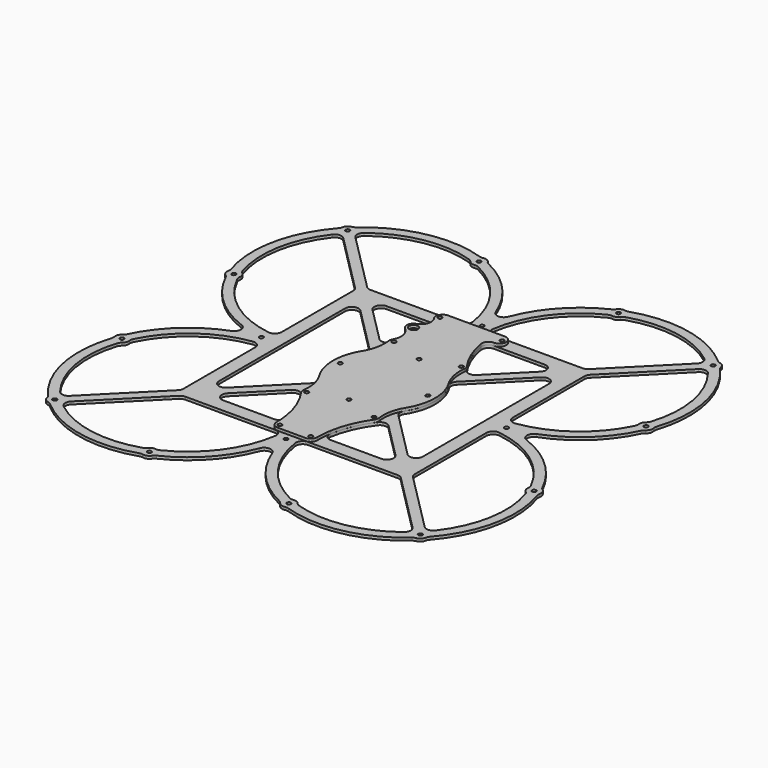
from build123d import *

# Parameters (mm, degrees)
F0_R     = 1.5
F0_W     = 52
F0_H     = 52
F1_DEPTH = 2
F2_R     = 1.5
F2_R_2   = 3.25
F3_DEPTH = 2
F4_D     = 3
F6_D     = 3


# Not quite as in the source:
# - a feature of the source that left no trace in its solid (it failed there, or was rolled back) is left out
# - a feature names something its author has since deleted; it is built from what else it names


with BuildPart() as f1:
    # F0 (on Top) → F1 (new body)
    with BuildSketch(Plane.XY):
        with BuildLine():
            ThreePointArc((-4.6783625731, -108.4060017484), (0, -105.1703496831), (4.6783625731, -108.4060017484))
            ThreePointArc((4.6783625731, -108.4060017484), (20.6623898882, -134.3994303851), (45.1726415045, -152.576202024))
            ThreePointArc((45.1726415045, -152.576202024), (46.2648777578, -153.2890175875), (47.1356036044, -154.2600595849))
            ThreePointArc((47.1356036044, -154.2600595849), (49.3956359115, -156.0747849076), (52.2827571645, -156.3307241522))
            ThreePointArc((52.2827571644, -156.3307241522), (53.5833623617, -156.2331937382), (54.8649423602, -156.4753481682))
            ThreePointArc((54.8649423602, -156.4753481682), (96.0251691017, -158.8888075411), (132.9814512389, -140.6070608479))
            ThreePointArc((132.9814512389, -140.6070608479), (134.0669737735, -139.8840623089), (135.3025491663, -139.4664027473))
            ThreePointArc((135.3025491663, -139.4664027473), (137.8609824083, -138.1042744963), (139.2338336739, -135.5515791701))
            ThreePointArc((139.2338336739, -135.5515791701), (139.656673946, -134.317767124), (140.3842208965, -133.2352877961))
            ThreePointArc((140.3842208965, -133.2352877961), (158.841500681, -96.2563147843), (156.5171132492, -54.9923735629))
            ThreePointArc((156.5171132492, -54.9923735629), (156.277094073, -53.7103919501), (156.3767909626, -52.4099510283))
            ThreePointArc((156.3767909626, -52.4099510283), (156.1256615791, -49.5224074254), (154.3147036453, -47.2593551971))
            ThreePointArc((154.3147036453, -47.2593551971), (153.3451134924, -46.38701295), (152.6341184178, -45.2935907696))
            ThreePointArc((152.6341184178, -45.2935907696), (134.44883526, -20.7077210858), (108.4060017484, -4.6783625731))
            ThreePointArc((108.4060017484, -4.6783625731), (105.1703496831, 0), (108.4060017484, 4.6783625731))
            ThreePointArc((108.4060017484, 4.6783625731), (134.44883526, 20.7077210858), (152.6341184178, 45.2935907696))
            ThreePointArc((152.6341184178, 45.2935907696), (153.3451134924, 46.38701295), (154.3147036453, 47.2593551971))
            ThreePointArc((154.3147036453, 47.2593551971), (156.1256615791, 49.5224074254), (156.3767909626, 52.4099510283))
            ThreePointArc((156.3767909626, 52.4099510283), (156.277094073, 53.7103919501), (156.5171132492, 54.9923735629))
            ThreePointArc((156.5171132492, 54.9923735629), (158.841500681, 96.2563147843), (140.3842208965, 133.2352877961))
            ThreePointArc((140.3842208965, 133.2352877961), (139.656673946, 134.317767124), (139.2338336739, 135.5515791701))
            ThreePointArc((139.2338336739, 135.5515791701), (137.8609824083, 138.1042744963), (135.3025491663, 139.4664027473))
            ThreePointArc((135.3025491663, 139.4664027473), (134.0669737735, 139.8840623089), (132.9814512389, 140.6070608479))
            ThreePointArc((132.9814512389, 140.6070608479), (96.0251691017, 158.8888075411), (54.8649423602, 156.4753481682))
            ThreePointArc((54.8649423602, 156.4753481682), (53.5833623617, 156.2331937382), (52.2827571645, 156.3307241522))
            ThreePointArc((52.2827571645, 156.3307241522), (49.3956359115, 156.0747849076), (47.1356036044, 154.2600595849))
            ThreePointArc((47.1356036044, 154.2600595849), (46.2648777578, 153.2890175875), (45.1726415045, 152.576202024))
            ThreePointArc((45.1726415045, 152.576202024), (20.6623898883, 134.3994303851), (4.6783625731, 108.4060017484))
            ThreePointArc((4.6783625731, 108.4060017484), (0, 105.1703496831), (-4.6783625731, 108.4060017484))
            ThreePointArc((-4.6783625731, 108.4060017484), (-20.6623898882, 134.3994303851), (-45.1726415045, 152.576202024))
            ThreePointArc((-45.1726415045, 152.576202024), (-46.2648777578, 153.2890175875), (-47.1356036044, 154.2600595849))
            ThreePointArc((-47.1356036044, 154.2600595849), (-49.3956359115, 156.0747849076), (-52.2827571644, 156.3307241522))
            ThreePointArc((-52.2827571644, 156.3307241522), (-53.5833623617, 156.2331937382), (-54.8649423602, 156.4753481682))
            ThreePointArc((-54.8649423602, 156.4753481682), (-96.0251691017, 158.8888075411), (-132.9814512389, 140.6070608479))
            ThreePointArc((-132.9814512389, 140.6070608479), (-134.0669737735, 139.8840623089), (-135.3025491663, 139.4664027473))
            ThreePointArc((-135.3025491663, 139.4664027473), (-137.8609824083, 138.1042744963), (-139.2338336739, 135.5515791701))
            ThreePointArc((-139.2338336739, 135.5515791701), (-139.656673946, 134.317767124), (-140.3842208964, 133.2352877961))
            ThreePointArc((-140.3842208964, 133.2352877961), (-158.841500681, 96.2563147843), (-156.5171132492, 54.9923735629))
            ThreePointArc((-156.5171132492, 54.9923735629), (-156.277094073, 53.7103919501), (-156.3767909626, 52.4099510283))
            ThreePointArc((-156.3767909626, 52.4099510283), (-156.1256615791, 49.5224074254), (-154.3147036453, 47.2593551971))
            ThreePointArc((-154.3147036453, 47.2593551971), (-153.3451134924, 46.38701295), (-152.6341184178, 45.2935907696))
            ThreePointArc((-152.6341184178, 45.2935907696), (-134.44883526, 20.7077210858), (-108.4060017484, 4.6783625731))
            ThreePointArc((-108.4060017484, 4.6783625731), (-105.1703496831, 0), (-108.4060017484, -4.6783625731))
            ThreePointArc((-108.4060017484, -4.6783625731), (-134.44883526, -20.7077210858), (-152.6341184178, -45.2935907696))
            ThreePointArc((-152.6341184178, -45.2935907696), (-153.3451134924, -46.38701295), (-154.3147036453, -47.2593551971))
            ThreePointArc((-154.3147036453, -47.2593551971), (-156.1256615791, -49.5224074254), (-156.3767909626, -52.4099510283))
            ThreePointArc((-156.3767909626, -52.4099510283), (-156.277094073, -53.7103919501), (-156.5171132492, -54.9923735629))
            ThreePointArc((-156.5171132492, -54.9923735629), (-158.841500681, -96.2563147843), (-140.3842208965, -133.2352877961))
            ThreePointArc((-140.3842208965, -133.2352877961), (-139.656673946, -134.317767124), (-139.2338336739, -135.5515791701))
            ThreePointArc((-139.2338336739, -135.5515791701), (-137.8609824083, -138.1042744963), (-135.3025491663, -139.4664027473))
            ThreePointArc((-135.3025491663, -139.4664027473), (-134.0669737735, -139.8840623089), (-132.9814512389, -140.6070608479))
            ThreePointArc((-132.9814512389, -140.6070608479), (-96.0251691017, -158.8888075411), (-54.8649423602, -156.4753481682))
            ThreePointArc((-54.8649423602, -156.4753481682), (-53.5833623617, -156.2331937382), (-52.2827571644, -156.3307241522))
            ThreePointArc((-52.2827571644, -156.3307241522), (-49.3956359115, -156.0747849076), (-47.1356036044, -154.2600595849))
            ThreePointArc((-47.1356036044, -154.2600595849), (-46.2648777578, -153.2890175875), (-45.1726415045, -152.576202024))
            ThreePointArc((-45.1726415045, -152.576202024), (-20.6623898883, -134.3994303851), (-4.6783625731, -108.4060017484))
        make_face()
        with Locations((-134.3328737249, -134.5613309295)):
            Circle(F0_R, mode=Mode.SUBTRACT)
        with Locations((-51.261755673, -151.4360785108)):
            Circle(F0_R, mode=Mode.SUBTRACT)
        with BuildLine():
            Line((-63.8445055786, -85), (-12.2338580115, -85))
            ThreePointArc((-12.2338580115, -85), (-8.449043945, -86.7327102238), (-7.2874242898, -90.7299270073))
            ThreePointArc((-7.2874242898, -90.7299270073), (-20.6592480643, -123.369634074), (-47.6974444383, -146.0211701213))
            ThreePointArc((-47.6974444383, -146.0211701213), (-49.1034491788, -146.4668977038), (-50.5783264353, -146.4830062847))
            ThreePointArc((-50.5783264353, -146.4830062847), (-53.1278754345, -146.797372114), (-55.1848415227, -148.3361757032))
            ThreePointArc((-55.1848415227, -148.3361757032), (-56.2599847868, -149.3459228844), (-57.5829585674, -149.9980446399))
            ThreePointArc((-57.5829585674, -149.9980446399), (-92.774950649, -152.3812865036), (-125.0248290935, -138.0948772707))
            ThreePointArc((-125.0248290935, -138.0948772707), (-126.9516515098, -134.4630557485), (-125.5048591166, -130.6147361199))
            Line((-125.5048591166, -130.6147361199), (-89.5414765929, -94.500135866))
            Line((-89.5414765929, -94.500135866), (-87.4194344398, -92.369171015))
            Line((-87.4194344398, -92.369171015), (-87.1110934803, -92.0595335529))
            Line((-87.1110934803, -92.0595335529), (-81.5468476147, -86.4718913166))
            ThreePointArc((-81.5468476147, -86.4718913166), (-79.9221658369, -85.3826120253), (-78.0039040479, -85))
            Line((-78.0039040479, -85), (-63.8445055786, -85))
        make_face(mode=Mode.SUBTRACT)
        with Locations((0, -90.0851748435)):
            Circle(F0_R, mode=Mode.SUBTRACT)
        with Locations((-151.4838529462, -51.3807972166)):
            Circle(F0_R, mode=Mode.SUBTRACT)
        with BuildLine():
            Line((-85, -12.2338580115), (-85, -63.8445055786))
            Line((-85, -63.8445055786), (-85, -77.954308432))
            ThreePointArc((-85, -77.954308432), (-85.3785977326, -79.8628788611), (-86.4570564332, -81.4824171154))
            Line((-86.4570564332, -81.4824171154), (-92.0605119902, -87.1094339109))
            Line((-92.0605119902, -87.1094339109), (-92.3795554334, -87.4298188582))
            Line((-92.3795554334, -87.4298188582), (-94.4808633591, -89.5399622991))
            Line((-94.4808633591, -89.5399622991), (-130.4597965625, -125.6701786198))
            ThreePointArc((-130.4597965625, -125.6701786198), (-134.3041683832, -127.1329757667), (-137.9445459782, -125.2181334353))
            ThreePointArc((-137.9445459782, -125.2181334353), (-152.3491388582, -92.9557750243), (-150.0352909057, -57.6995957938))
            ThreePointArc((-150.0352909057, -57.6995957938), (-149.3853739286, -56.375537513), (-148.3774191741, -55.2987136551))
            ThreePointArc((-148.3774191741, -55.2987136551), (-146.8420443134, -53.2391870077), (-146.5319260821, -50.6891178603))
            ThreePointArc((-146.5319260821, -50.6891178603), (-146.5182744452, -49.2142158157), (-146.0748896718, -47.8074705116))
            ThreePointArc((-146.0748896718, -47.8074705116), (-123.4190453917, -20.6953922762), (-90.7299270073, -7.2874242898))
            ThreePointArc((-90.7299270073, -7.2874242898), (-86.7327102238, -8.449043945), (-85, -12.2338580115))
        make_face(mode=Mode.SUBTRACT)
        with BuildLine():
            Line((-20.8392021683, -75.0000000042), (-51.3047130828, -75.0000000043))
            Line((-51.3047130828, -75.0000000043), (-58.0876473189, -75.0000000043))
            ThreePointArc((-58.0876473189, -75.0000000043), (-62.7050352935, -71.9182617933), (-61.6305908857, -66.4718913208))
            Line((-61.6305908857, -66.4718913208), (-35.6274832487, -40.3594466126))
            ThreePointArc((-35.6274832487, -40.3594466126), (-31.7411740863, -38.8993592225), (-28.0915846553, -40.8781849041))
            ThreePointArc((-28.0915846553, -40.8781849041), (-20.3006049384, -54.2904253384), (-15.9091356823, -69.1666666712))
            ThreePointArc((-15.9091356823, -69.1666666712), (-17.0203890893, -73.2274861262), (-20.8392021683, -75.0000000042))
        make_face(mode=Mode.SUBTRACT)
        with BuildLine():
            Line((-75.0000000043, -57.8702130484), (-75.0000000043, -51.3047130828))
            Line((-75.0000000043, -51.3047130828), (-75.000000004, 51.3047130826))
            Line((-75.000000004, 51.3047130826), (-75.000000004, 57.8702130481))
            ThreePointArc((-75.000000004, 57.8702130481), (-71.9085704331, 62.4916153155), (-66.4570564372, 61.3983217315))
            Line((-66.4570564372, 61.3983217315), (-32.013039726, 26.809475873))
            ThreePointArc((-32.013039726, 26.809475873), (-30.5818618176, 23.7894179246), (-31.372926442, 20.542382819))
            ThreePointArc((-31.372926442, 20.542382819), (-32.5112791832, 18.688679228), (-33.540230714, 16.7720877968))
            ThreePointArc((-33.540230714, 16.7720877968), (-37.5000000722, 0), (-33.540230714, -16.7720877968))
            ThreePointArc((-33.540230714, -16.7720877968), (-32.5112791832, -18.688679228), (-31.3729264419, -20.542382819))
            ThreePointArc((-31.3729264419, -20.542382819), (-30.5818618175, -23.7894179247), (-32.013039726, -26.8094758731))
            Line((-32.013039726, -26.8094758731), (-66.4570564374, -61.3983217318))
            ThreePointArc((-66.4570564374, -61.3983217318), (-71.9085704334, -62.4916153158), (-75.0000000043, -57.8702130484))
        make_face(mode=Mode.SUBTRACT)
        with Locations((0, -32.2011839358)):
            Circle(F0_R, mode=Mode.SUBTRACT)
        with Locations((51.261755673, -151.4360785108)):
            Circle(F0_R, mode=Mode.SUBTRACT)
        with BuildLine():
            Line((12.2338580115, -85), (63.8445055786, -85))
            Line((63.8445055786, -85), (78.0039040479, -85))
            ThreePointArc((78.0039040479, -85), (79.9221658369, -85.3826120253), (81.5468476147, -86.4718913166))
            Line((81.5468476147, -86.4718913166), (87.1110934804, -92.0595335529))
            Line((87.1110934803, -92.0595335529), (87.4194344398, -92.369171015))
            Line((87.4194344398, -92.369171015), (89.5414765929, -94.500135866))
            Line((89.5414765929, -94.500135866), (125.5048591166, -130.6147361199))
            ThreePointArc((125.5048591166, -130.6147361199), (126.9516515098, -134.4630557485), (125.0248290936, -138.0948772707))
            ThreePointArc((125.0248290936, -138.0948772707), (92.774950649, -152.3812865036), (57.5829585673, -149.9980446399))
            ThreePointArc((57.5829585673, -149.9980446399), (56.2599847868, -149.3459228844), (55.1848415227, -148.3361757032))
            ThreePointArc((55.1848415227, -148.3361757032), (53.1278754345, -146.797372114), (50.5783264353, -146.4830062847))
            ThreePointArc((50.5783264353, -146.4830062847), (49.1034491788, -146.4668977038), (47.6974444383, -146.0211701213))
            ThreePointArc((47.6974444383, -146.0211701213), (20.6592480643, -123.369634074), (7.2874242897, -90.7299270073))
            ThreePointArc((7.2874242897, -90.7299270073), (8.449043945, -86.7327102238), (12.2338580115, -85))
        make_face(mode=Mode.SUBTRACT)
        with Locations((134.3328737249, -134.5613309295)):
            Circle(F0_R, mode=Mode.SUBTRACT)
        with BuildLine():
            Line((58.0876473187, -75.000000004), (51.3047130826, -75.000000004))
            Line((51.3047130826, -75.000000004), (20.8392021683, -75.0000000041))
            ThreePointArc((20.8392021683, -75.0000000041), (17.0203890893, -73.2274861261), (15.9091356823, -69.1666666711))
            ThreePointArc((15.9091356823, -69.1666666711), (20.3006049384, -54.2904253384), (28.0915846553, -40.878184904))
            ThreePointArc((28.0915846553, -40.878184904), (31.7411740863, -38.8993592225), (35.6274832487, -40.3594466126))
            Line((35.6274832487, -40.3594466126), (61.6305908855, -66.4718913206))
            ThreePointArc((61.6305908855, -66.4718913206), (62.7050352933, -71.9182617931), (58.0876473187, -75.000000004))
        make_face(mode=Mode.SUBTRACT)
        with BuildLine():
            Line((85, -77.9543084319), (85, -63.8445055786))
            Line((85, -63.8445055786), (85, -12.2338580115))
            ThreePointArc((85, -12.2338580115), (86.7327102238, -8.449043945), (90.7299270073, -7.2874242898))
            ThreePointArc((90.7299270073, -7.2874242898), (123.4190453917, -20.6953922762), (146.0748896718, -47.8074705116))
            ThreePointArc((146.0748896718, -47.8074705116), (146.5182744452, -49.2142158157), (146.5319260821, -50.6891178603))
            ThreePointArc((146.5319260821, -50.6891178603), (146.8420443134, -53.2391870077), (148.3774191741, -55.298713655))
            ThreePointArc((148.3774191741, -55.2987136551), (149.3853739286, -56.375537513), (150.0352909057, -57.6995957938))
            ThreePointArc((150.0352909057, -57.6995957938), (152.3491388582, -92.9557750243), (137.9445459782, -125.2181334353))
            ThreePointArc((137.9445459782, -125.2181334353), (134.3041683832, -127.1329757667), (130.4597965625, -125.6701786198))
            Line((130.4597965625, -125.6701786198), (94.4808633591, -89.5399622991))
            Line((94.4808633591, -89.5399622991), (92.3795554334, -87.4298188582))
            Line((92.3795554334, -87.4298188582), (92.0605119902, -87.1094339109))
            Line((92.0605119902, -87.1094339109), (86.4570564331, -81.4824171154))
            ThreePointArc((86.4570564331, -81.4824171154), (85.3785977326, -79.8628788611), (85, -77.9543084319))
        make_face(mode=Mode.SUBTRACT)
        with Locations((151.4838529462, -51.3807972166)):
            Circle(F0_R, mode=Mode.SUBTRACT)
        with Locations((-90.0851748436, 0)):
            Circle(F0_R, mode=Mode.SUBTRACT)
        with Locations((-151.4838529462, 51.3807972166)):
            Circle(F0_R, mode=Mode.SUBTRACT)
        with BuildLine():
            Line((-85, 63.8445055786), (-85, 12.2338580115))
            ThreePointArc((-85, 12.2338580115), (-86.7327102238, 8.449043945), (-90.7299270073, 7.2874242898))
            ThreePointArc((-90.7299270073, 7.2874242898), (-123.4190453917, 20.6953922762), (-146.0748896718, 47.8074705116))
            ThreePointArc((-146.0748896718, 47.8074705116), (-146.5182744452, 49.2142158157), (-146.5319260821, 50.6891178603))
            ThreePointArc((-146.5319260821, 50.6891178603), (-146.8420443134, 53.2391870077), (-148.3774191741, 55.2987136551))
            ThreePointArc((-148.3774191741, 55.2987136551), (-149.3853739286, 56.375537513), (-150.0352909057, 57.6995957938))
            ThreePointArc((-150.0352909057, 57.6995957938), (-152.3491388582, 92.9557750243), (-137.9445459782, 125.2181334353))
            ThreePointArc((-137.9445459782, 125.2181334353), (-134.3041683832, 127.1329757667), (-130.4597965625, 125.6701786198))
            Line((-130.4597965625, 125.6701786198), (-94.4808633591, 89.5399622991))
            Line((-94.4808633591, 89.5399622991), (-92.3795554334, 87.4298188582))
            Line((-92.3795554334, 87.4298188582), (-92.0605119902, 87.1094339109))
            Line((-92.0605119902, 87.1094339109), (-86.4570564331, 81.4824171154))
            ThreePointArc((-86.4570564331, 81.4824171154), (-85.3785977326, 79.8628788611), (-85, 77.9543084319))
            Line((-85, 77.9543084319), (-85, 63.8445055786))
        make_face(mode=Mode.SUBTRACT)
        with Locations((-32.1965969132, 0)):
            Circle(F0_R, mode=Mode.SUBTRACT)
        Rectangle(F0_W, F0_H, mode=Mode.SUBTRACT)
        with Locations((0, 32.2011839358)):
            Circle(F0_R, mode=Mode.SUBTRACT)
        with BuildLine():
            Line((-58.0876473187, 75.000000004), (-51.3047130826, 75.000000004))
            Line((-51.3047130826, 75.000000004), (-20.8392021683, 75.000000004))
            ThreePointArc((-20.8392021683, 75.000000004), (-17.0203890893, 73.2274861259), (-15.9091356824, 69.1666666709))
            ThreePointArc((-15.9091356824, 69.1666666709), (-20.3006049385, 54.2904253383), (-28.0915846553, 40.878184904))
            ThreePointArc((-28.0915846553, 40.878184904), (-31.7411740863, 38.8993592225), (-35.6274832487, 40.3594466126))
            Line((-35.6274832487, 40.3594466126), (-61.6305908855, 66.4718913206))
            ThreePointArc((-61.6305908855, 66.4718913206), (-62.7050352934, 71.9182617931), (-58.0876473187, 75.000000004))
        make_face(mode=Mode.SUBTRACT)
        with Locations((-134.3328737249, 134.5613309295)):
            Circle(F0_R, mode=Mode.SUBTRACT)
        with BuildLine():
            ThreePointArc((-7.2874242898, 90.7299270073), (-8.449043945, 86.7327102238), (-12.2338580115, 85))
            Line((-12.2338580115, 85), (-63.8445055786, 85))
            Line((-63.8445055786, 85), (-78.0039040479, 85))
            ThreePointArc((-78.0039040479, 85), (-79.922165837, 85.3826120254), (-81.5468476148, 86.4718913166))
            Line((-81.5468476148, 86.4718913166), (-87.1110934804, 92.0595335529))
            Line((-87.1110934803, 92.0595335529), (-87.4194344398, 92.369171015))
            Line((-87.4194344398, 92.369171015), (-89.5414765929, 94.500135866))
            Line((-89.5414765929, 94.500135866), (-125.5048591166, 130.6147361199))
            ThreePointArc((-125.5048591166, 130.6147361199), (-126.9516515098, 134.4630557485), (-125.0248290936, 138.0948772707))
            ThreePointArc((-125.0248290936, 138.0948772707), (-92.774950649, 152.3812865036), (-57.5829585674, 149.9980446399))
            ThreePointArc((-57.5829585674, 149.9980446399), (-56.2599847868, 149.3459228844), (-55.1848415227, 148.3361757032))
            ThreePointArc((-55.1848415227, 148.3361757032), (-53.1278754345, 146.797372114), (-50.5783264353, 146.4830062847))
            ThreePointArc((-50.5783264353, 146.4830062847), (-49.1034491788, 146.4668977038), (-47.6974444383, 146.0211701213))
            ThreePointArc((-47.6974444383, 146.0211701213), (-20.6592480643, 123.369634074), (-7.2874242898, 90.7299270073))
        make_face(mode=Mode.SUBTRACT)
        with Locations((0, 90.0851748435)):
            Circle(F0_R, mode=Mode.SUBTRACT)
        with Locations((-51.261755673, 151.4360785108)):
            Circle(F0_R, mode=Mode.SUBTRACT)
        with Locations((32.1965969132, 0)):
            Circle(F0_R, mode=Mode.SUBTRACT)
        with BuildLine():
            Line((75.0000273885, 51.3041211149), (74.9999753624, -51.3429242195))
            Line((74.9999753624, -51.3429242195), (74.9999753624, -57.8701883029))
            ThreePointArc((74.9999753624, -57.8701883029), (71.9085457915, -62.4915905703), (66.4570317955, -61.3982969863))
            Line((66.4570317955, -61.3982969863), (32.013039726, -26.8094758731))
            ThreePointArc((32.013039726, -26.8094758731), (30.5818618175, -23.7894179247), (31.3729264419, -20.542382819))
            ThreePointArc((31.3729264419, -20.542382819), (32.5089467844, -18.6927361396), (33.5360437181, -16.7804581926))
            ThreePointArc((33.5360437181, -16.7804581926), (37.4999996469, -0.0056476077), (33.5410965671, 16.7703561826))
            ThreePointArc((33.5410965671, 16.7703561826), (32.5117615955, 18.6878399869), (31.3729264419, 20.5423828191))
            ThreePointArc((31.3729264419, 20.5423828191), (30.5818618175, 23.7894179247), (32.0130397259, 26.8094758731))
            Line((32.0130397259, 26.8094758731), (66.4570838216, 61.3983492312))
            ThreePointArc((66.4570838216, 61.3983492312), (71.9085978176, 62.4916428152), (75.0000273885, 57.8702405478))
            Line((75.0000273885, 57.8702405478), (75.0000273885, 51.3041211149))
        make_face(mode=Mode.SUBTRACT)
        with BuildLine():
            Line((20.8392021684, 75.0000000039), (51.3047130824, 75.0000000038))
            Line((51.3047130824, 75.0000000038), (58.0876473184, 75.0000000038))
            ThreePointArc((58.0876473184, 75.0000000038), (62.7050352931, 71.9182617929), (61.6305908852, 66.4718913204))
            Line((61.6305908852, 66.4718913204), (35.6274832486, 40.3594466126))
            ThreePointArc((35.6274832486, 40.3594466126), (31.7411740862, 38.8993592226), (28.0915846553, 40.8781849041))
            ThreePointArc((28.0915846553, 40.8781849041), (20.3006049385, 54.2904253383), (15.9091356824, 69.1666666709))
            ThreePointArc((15.9091356824, 69.1666666709), (17.0203890893, 73.2274861258), (20.8392021684, 75.0000000039))
        make_face(mode=Mode.SUBTRACT)
        with Locations((90.0851748436, 0)):
            Circle(F0_R, mode=Mode.SUBTRACT)
        with BuildLine():
            ThreePointArc((90.7299270073, 7.2874242898), (86.7327102238, 8.449043945), (85, 12.2338580115))
            Line((85, 12.2338580115), (85, 63.8445055786))
            Line((85, 63.8445055786), (85, 77.954308432))
            ThreePointArc((85, 77.954308432), (85.3785977326, 79.8628788611), (86.4570564331, 81.4824171154))
            Line((86.4570564331, 81.4824171154), (92.0605119902, 87.1094339109))
            Line((92.0605119902, 87.1094339109), (92.3795554334, 87.4298188582))
            Line((92.3795554334, 87.4298188582), (94.4808633591, 89.5399622991))
            Line((94.4808633591, 89.5399622991), (130.4597965625, 125.6701786198))
            ThreePointArc((130.4597965625, 125.6701786198), (134.3041683832, 127.1329757667), (137.9445459782, 125.2181334353))
            ThreePointArc((137.9445459782, 125.2181334353), (152.3491388582, 92.9557750243), (150.0352909057, 57.6995957938))
            ThreePointArc((150.0352909057, 57.6995957938), (149.3853739286, 56.375537513), (148.3774191741, 55.2987136551))
            ThreePointArc((148.3774191741, 55.2987136551), (146.8420443134, 53.2391870077), (146.5319260821, 50.6891178603))
            ThreePointArc((146.5319260821, 50.6891178603), (146.5182744452, 49.2142158157), (146.0748896718, 47.8074705116))
            ThreePointArc((146.0748896718, 47.8074705116), (123.4190453917, 20.6953922762), (90.7299270073, 7.2874242897))
        make_face(mode=Mode.SUBTRACT)
        with Locations((151.4838529462, 51.3807972166)):
            Circle(F0_R, mode=Mode.SUBTRACT)
        with BuildLine():
            Line((78.0039040478, 85), (63.8445055786, 85))
            Line((63.8445055786, 85), (12.2338580115, 85))
            ThreePointArc((12.2338580115, 85), (8.449043945, 86.7327102238), (7.2874242898, 90.7299270073))
            ThreePointArc((7.2874242898, 90.7299270073), (20.6592480643, 123.369634074), (47.6974444383, 146.0211701213))
            ThreePointArc((47.6974444383, 146.0211701213), (49.1034491788, 146.4668977038), (50.5783264353, 146.4830062847))
            ThreePointArc((50.5783264353, 146.4830062847), (53.1278754345, 146.797372114), (55.1848415227, 148.3361757032))
            ThreePointArc((55.1848415227, 148.3361757032), (56.2599847868, 149.3459228844), (57.5829585674, 149.9980446399))
            ThreePointArc((57.5829585674, 149.9980446399), (92.774950649, 152.3812865036), (125.0248290935, 138.0948772707))
            ThreePointArc((125.0248290935, 138.0948772707), (126.9516515098, 134.4630557485), (125.5048591166, 130.6147361199))
            Line((125.5048591166, 130.6147361199), (89.5414765929, 94.500135866))
            Line((89.5414765929, 94.500135866), (87.4194344398, 92.369171015))
            Line((87.4194344398, 92.369171015), (87.1110934803, 92.0595335529))
            Line((87.1110934803, 92.0595335529), (81.5468476147, 86.4718913165))
            ThreePointArc((81.5468476147, 86.4718913165), (79.9221658369, 85.3826120253), (78.0039040478, 85))
        make_face(mode=Mode.SUBTRACT)
        with Locations((51.261755673, 151.4360785108)):
            Circle(F0_R, mode=Mode.SUBTRACT)
        with Locations((134.3328737249, 134.5613309295)):
            Circle(F0_R, mode=Mode.SUBTRACT)
        Rectangle(F0_W, F0_H)
        with Locations((-15.25, -15.25)):
            Circle(F0_R, mode=Mode.SUBTRACT)
        with Locations((15.25, -15.25)):
            Circle(F0_R, mode=Mode.SUBTRACT)
        with Locations((-15.25, 15.25)):
            Circle(F0_R, mode=Mode.SUBTRACT)
        with Locations((15.25, 15.25)):
            Circle(F0_R, mode=Mode.SUBTRACT)
    extrude(amount=F1_DEPTH)

    # F4 (through all)
    with Locations(Plane.XY.offset(2)):
        with Locations((-22.8392021664, 80.000000002), (22.8392021664, 80.000000002), (24.762961832, 40.1063807227), (-24.762961832, 40.1063807227), (24.762961832, -40.1063807227), (-24.762961832, -40.1063807227), (11.3338878595, -81.490215816), (-11.3338878595, -81.490215816)):
            Hole(F4_D / 2)


with BuildPart() as f3:
    # F2 (on face) → F3 (new body)
    with BuildSketch(Plane.XY.offset(2)):
        with BuildLine():
            ThreePointArc((-15.9091356824, 69.1666666709), (-19.9106965579, 55.2154158428), (-26.9081876363, 42.4998738677))
            ThreePointArc((-26.9081876363, 42.4998738677), (-27.6769238616, 40.8198612546), (-27.7830892982, 38.9753757804))
            ThreePointArc((-27.7830892982, 38.9753757804), (-28.007128425, 29.9078433424), (-30.9528290829, 21.3291962649))
            ThreePointArc((-30.9528290829, 21.3291962649), (-31.1452979661, 20.9264032941), (-31.372926442, 20.542382819))
            ThreePointArc((-31.372926442, 20.542382819), (-31.4056737141, 20.4922830348), (-31.4383409814, 20.4421310472))
            ThreePointArc((-31.4383409814, 20.4421310472), (-31.6830287788, 20.0206330091), (-31.9345881999, 19.6031996946))
            ThreePointArc((-31.9345881999, 19.6031996946), (-37.4713152243, -0.0624269617), (-31.8690935102, -19.7094962036))
            ThreePointArc((-31.8690935102, -19.7094962036), (-31.6175512894, -20.1238791031), (-31.3729264419, -20.542382819))
            ThreePointArc((-31.3729264419, -20.542382819), (-31.1884956627, -20.8472242602), (-31.0262417656, -21.1644255992))
            ThreePointArc((-31.0262417656, -21.1644255992), (-27.9828775906, -29.8047077735), (-27.7678949187, -38.9627820254))
            ThreePointArc((-27.7678949187, -38.9627820254), (-27.669162447, -40.8212491731), (-26.8976008529, -42.5148668827))
            ThreePointArc((-26.8976008529, -42.5148668827), (-19.9071979487, -55.2238997898), (-15.9091356823, -69.1666666712))
            ThreePointArc((-15.9091356823, -69.1666666712), (-15.2276826852, -74.5642930841), (-15, -80))
            ThreePointArc((-15, -80), (-13.5355339059, -83.5355339059), (-10, -85))
            Line((-10, -85), (10, -85))
            ThreePointArc((10, -85), (13.5355339059, -83.5355339059), (15, -80))
            ThreePointArc((15, -80), (15.2276826852, -74.5642930841), (15.9091356823, -69.1666666711))
            ThreePointArc((15.9091356823, -69.1666666711), (19.9017495941, -55.237118541), (26.8811153584, -42.5382315629))
            ThreePointArc((26.8811153584, -42.5382315629), (27.6569591075, -40.8235247898), (27.7439374691, -38.9434748955))
            ThreePointArc((27.7439374691, -38.9434748955), (28.0647603863, -29.0510560979), (31.7678464213, -19.8722745431))
            ThreePointArc((31.7678464213, -19.8722745431), (37.4701194039, -0.3057999751), (32.0879553062, 19.3511365566))
            ThreePointArc((32.0879553062, 19.3511365566), (31.8364128835, 19.7758153076), (31.5916311201, 20.2044264602))
            ThreePointArc((31.5916311201, 20.2044264602), (31.482732265, 20.3736981067), (31.3729264419, 20.5423828191))
            ThreePointArc((31.3729264419, 20.5423828191), (31.0658902061, 21.0815799107), (30.8280022576, 21.6546541446))
            ThreePointArc((30.8280022576, 21.6546541446), (28.0712651547, 30.112763477), (27.8177487263, 39.0051727316))
            ThreePointArc((27.8177487263, 39.0051727316), (27.694698691, 40.8168605911), (26.9327469567, 42.4651274888))
            ThreePointArc((26.9327469567, 42.4651274888), (19.9188118912, 55.1957496498), (15.9091356824, 69.1666666709))
            ThreePointArc((15.9091356824, 69.1666666709), (17.0203890893, 73.2274861258), (20.8392021684, 75.0000000039))
            ThreePointArc((20.8392021684, 75.0000000039), (25.8392021663, 80.0000000019), (20.8392021684, 84.9999999999))
            Line((20.8392021684, 84.9999999999), (12.2338580115, 84.9999999999))
            Line((12.2338580115, 84.9999999999), (10, 84.9999999999))
            Line((10, 85), (-10, 85))
            Line((-10, 85), (-12.2338580115, 85))
            Line((-12.2338580115, 85), (-20.8392021683, 85))
            ThreePointArc((-20.8392021683, 85), (-25.2890194103, 82.2801593152), (-24.8977190605, 77.0796506023))
            ThreePointArc((-24.8977190605, 77.0796506023), (-23.1193614816, 75.55018276), (-20.8392021683, 75.000000004))
            ThreePointArc((-20.8392021683, 75.000000004), (-17.0203890893, 73.2274861259), (-15.9091356824, 69.1666666709))
        make_face()
        with Locations((-11.3338878595, -81.490215816)):
            Circle(F2_R, mode=Mode.SUBTRACT)
        with Locations((-24.762961832, -40.1063807227)):
            Circle(F2_R, mode=Mode.SUBTRACT)
        with Locations((0, -32.2011839358)):
            Circle(F2_R, mode=Mode.SUBTRACT)
        with Locations((-15.25, -15.25)):
            Circle(F2_R, mode=Mode.SUBTRACT)
        with Locations((11.3338878595, -81.490215816)):
            Circle(F2_R, mode=Mode.SUBTRACT)
        with Locations((24.762961832, -40.1063807227)):
            Circle(F2_R, mode=Mode.SUBTRACT)
        with Locations((15.25, -15.25)):
            Circle(F2_R, mode=Mode.SUBTRACT)
        with Locations((-32.1965969132, 0)):
            Circle(F2_R, mode=Mode.SUBTRACT)
        with Locations((-15.25, 15.25)):
            Circle(F2_R, mode=Mode.SUBTRACT)
        with Locations((-24.762961832, 40.1063807227)):
            Circle(F2_R, mode=Mode.SUBTRACT)
        with Locations((0, 32.2011839358)):
            Circle(F2_R, mode=Mode.SUBTRACT)
        with Locations((-22.8392021664, 80.000000002)):
            Circle(F2_R, mode=Mode.SUBTRACT)
        with Locations((15.25, 15.25)):
            Circle(F2_R, mode=Mode.SUBTRACT)
        with Locations((32.1965969132, 0)):
            Circle(F2_R, mode=Mode.SUBTRACT)
        with Locations((24.762961832, 40.1063807227)):
            Circle(F2_R, mode=Mode.SUBTRACT)
        with Locations((22.8392021664, 80.000000002)):
            Circle(F2_R, mode=Mode.SUBTRACT)
        with BuildLine():
            ThreePointArc((-30.0619339463, 56.9680733085), (-25.9181929267, 50.2934938027), (-26.9081876363, 42.4998738677))
            ThreePointArc((-26.9081876363, 42.4998738677), (-19.9106965579, 55.2154158428), (-15.9091356824, 69.1666666709))
            ThreePointArc((-15.9091356824, 69.1666666709), (-17.0203890893, 73.2274861259), (-20.8392021683, 75.000000004))
            Line((-20.8392021683, 75.000000004), (-23.843825872, 75.000000004))
            ThreePointArc((-23.843825872, 75.000000004), (-24.1093098285, 69.6236128094), (-27.8824838664, 65.7844490102))
            ThreePointArc((-27.8824838664, 65.7844490102), (-23.7553318557, 64.7282313694), (-21.9404339132, 60.8739967005))
            ThreePointArc((-21.9404339132, 60.8739967005), (-24.773350639, 56.3680284269), (-30.0619339463, 56.9680733085))
        make_face()
        with BuildLine():
            ThreePointArc((-27.8824838664, 65.7844490102), (-31.7943220198, 62.0739009672), (-30.0619339463, 56.9680733085))
            ThreePointArc((-30.0619339463, 56.9680733085), (-24.773350639, 56.3680284269), (-21.9404339132, 60.8739967005))
            ThreePointArc((-21.9404339132, 60.8739967005), (-23.7553318557, 64.7282313694), (-27.8824838664, 65.7844490102))
        make_face()
        with Locations((-26.9404339132, 60.8739967005)):
            Circle(F2_R_2, mode=Mode.SUBTRACT)
        with Locations((-15.25, 15.25)):
            Circle(F2_R)
        with Locations((15.25, 15.25)):
            Circle(F2_R)
        with Locations((32.1965969132, 0)):
            Circle(F2_R)
        with Locations((15.25, -15.25)):
            Circle(F2_R)
        with Locations((-15.25, -15.25)):
            Circle(F2_R)
        with BuildLine():
            Line((-23.843825872, 75.000000004), (-20.8392021683, 75.000000004))
            ThreePointArc((-20.8392021683, 75.000000004), (-23.1193614816, 75.55018276), (-24.8977190605, 77.0796506023))
            ThreePointArc((-24.8977190605, 77.0796506023), (-24.2901868849, 76.0806632186), (-23.843825872, 75.000000004))
        make_face()
    extrude(amount=F3_DEPTH)

    # F6 (through all)
    with Locations(Plane(origin=(0, 0, 0), x_dir=(1, 0, 0), z_dir=(0, 0, -1))):
        with Locations((0, 32.2011839358), (-32.1965969132, 0), (32.1965969132, 0), (0, -32.2011839358)):
            Hole(F6_D / 2)


solid = Compound([f1.part, f3.part])
